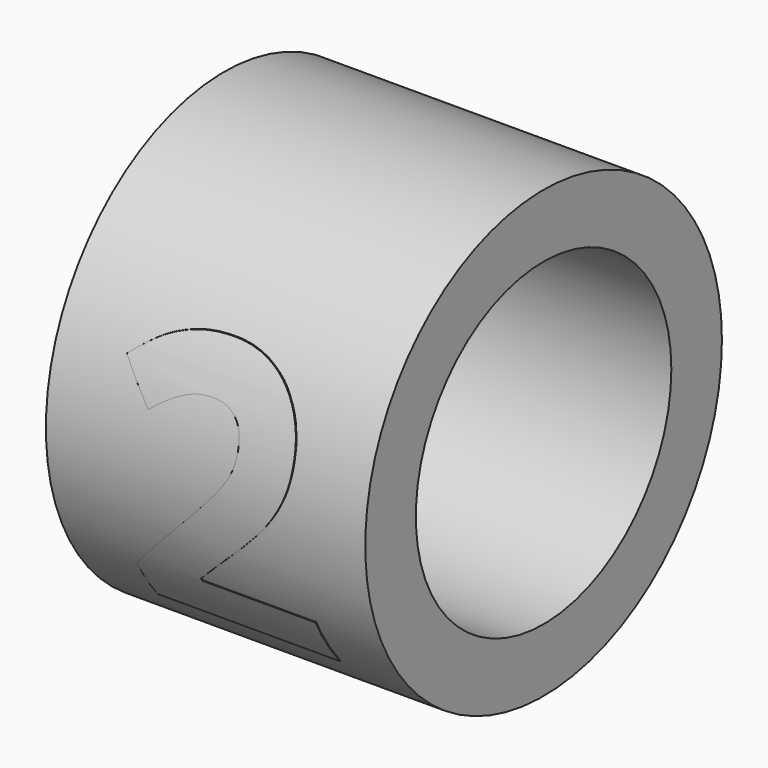
from build123d import *

# Parameters (mm, degrees)
F0_R         = 1.75
F0_R_2       = 1.745
F0_R_3       = 1.25
F1_DEPTH     = 2.5
F2_TEXT_SIZE = 2.8570699214
F3_REACH     = 4.2665280644
F4_DEPTH     = 2.5


# Not quite as in the source:
# - Text() gives the source's letters only with a copy of the font that has no kerning and outlines rounded to 1/6400 em; it was checked with that copy


with BuildPart() as f1:
    # F0 (on Right) → F1 (new body)
    with BuildSketch(Plane.YZ):
        Circle(F0_R)
        Circle(F0_R_2, mode=Mode.SUBTRACT)
        Circle(F0_R_2)
        Circle(F0_R_3, mode=Mode.SUBTRACT)
    extrude(amount=F1_DEPTH)

    f3_end = f1.faces().sort_by_distance((1.25, -1.75, 0))[0]
    # F2 (on Front) → F3 (intersect, up to a face of the model that its end follows)
    with BuildSketch(Plane.XZ):
        with Locations((0.4309935612, -1.1343103251)):
            Text('2', F2_TEXT_SIZE, font='Open Sans', font_style=FontStyle.BOLD, text_align=(TextAlign.LEFT, TextAlign.BOTTOM))
    f3_long = extrude(amount=F3_REACH, mode=Mode.PRIVATE)
    add(split(f3_long, bisect_by=f3_end, keep=Keep.BOTTOM, mode=Mode.PRIVATE), mode=Mode.INTERSECT)


with BuildPart() as f4:
    # F0 (on Right) → F4 (new body)
    with BuildSketch(Plane.YZ):
        Circle(F0_R_2)
        Circle(F0_R_3, mode=Mode.SUBTRACT)
    extrude(amount=F4_DEPTH)


solid = Compound([f1.part, f4.part])
